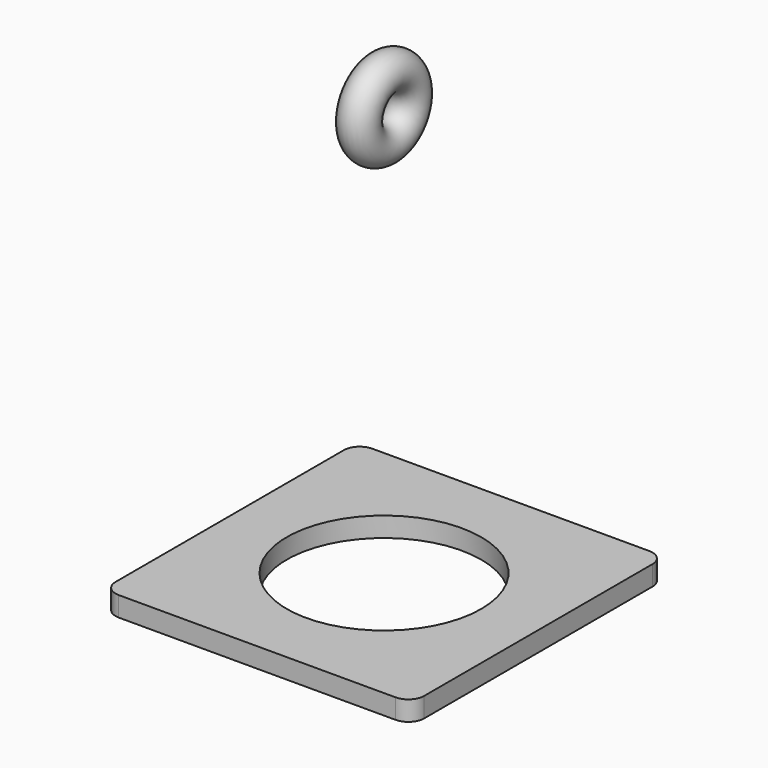
from build123d import *

# Parameters (mm, degrees)
F1_DEPTH = 1.5875
F4_R     = 1.445040765
F6_R     = 7.792593953
F7_DEPTH = 1.651


# Not quite as in the source:
# - the program builds the solid bodies; features that only make, move or delete a surface that nothing else refers to are left out


with BuildPart() as f1:
    # F0 (on Top) → F1 (new body)
    with BuildSketch(Plane.XY):
        with BuildLine():
            Line((-11.092720091, -12.7), (11.092720091, -12.7))
            ThreePointArc((11.092720091, -12.7), (11.9907457031, -12.3280256121), (12.362720091, -11.43))
            Line((12.362720091, -11.43), (12.362720091, 11.43))
            ThreePointArc((12.362720091, 11.43), (11.9907457031, 12.3280256121), (11.092720091, 12.7))
            Line((11.092720091, 12.7), (-11.092720091, 12.7))
            ThreePointArc((-11.092720091, 12.7), (-11.9907457031, 12.3280256121), (-12.362720091, 11.43))
            Line((-12.362720091, 11.43), (-12.362720091, -11.43))
            ThreePointArc((-12.362720091, -11.43), (-11.9907457031, -12.3280256121), (-11.092720091, -12.7))
        make_face()
    extrude(amount=F1_DEPTH)

    # F6 (on Top) → F7 (cut)
    with BuildSketch(Plane.XY):
        Circle(F6_R)
    extrude(amount=F7_DEPTH, mode=Mode.SUBTRACT)


with BuildPart() as f5:
    # F4 (on Front) → F5 (revolve)
    with BuildSketch(Plane.XZ):
        with Locations((0, 31.9377668202)):
            Circle(F4_R)
    revolve(axis=Axis((0.2411192982, 0, 34.4339795411), (1, 0, 0)))


solid = Compound([f1.part, f5.part])
